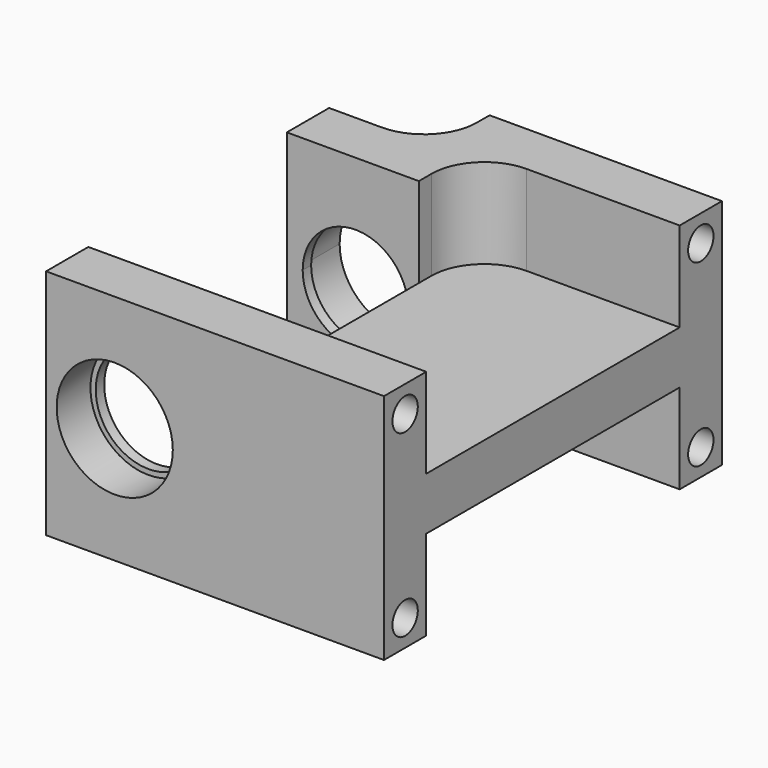
from build123d import *

# Parameters (mm, degrees)
F0_W      = 5
F0_H      = 5
F0_H_2    = 8.5
F0_W_2    = 30
F1_DEPTH  = 30
F2_DEPTH  = 2
F4_W      = 10.5
F4_H      = 30
F5_DEPTH  = 13.501
F3_R      = 5.5
F3_R_2    = 5
F3_R_3    = 2.5
F6_DEPTH  = 4
F7_DEPTH  = 5
F9_DEPTH  = 22
F10_DEPTH = 8
F11_DEPTH = 1.5
F12_R     = 5
F13_R     = 5
F15_DEPTH = 10.5
F14_R     = 2.5
F16_DEPTH = 11.5
F18_D     = 3
F20_D     = 2.5
F20_DEPTH = 15
F20_TIP   = 0.7510757738


# Not quite as in the source:
# - a feature names something its author has since deleted; it is built from what else it names


with BuildPart() as f1:
    # F0 (on Right) → F1 (new body)
    with BuildSketch(Plane.YZ):
        with Locations((17.5, 0)):
            Rectangle(F0_W, F0_H)
        with Locations((17.5, 6.75)):
            Rectangle(F0_W, F0_H_2)
        Rectangle(F0_W_2, F0_H)
        with Locations((17.5, -6.75)):
            Rectangle(F0_W, F0_H_2)
        with Locations((-17.5, 0)):
            Rectangle(F0_W, F0_H)
        with Locations((-17.5, 6.75)):
            Rectangle(F0_W, F0_H_2)
        with Locations((-17.5, -6.75)):
            Rectangle(F0_W, F0_H_2)
    extrude(amount=F1_DEPTH)

    # F0 (on Right) → F2 (join)
    with BuildSketch(Plane.YZ):
        with Locations((-17.5, 6.75)):
            Rectangle(F0_W, F0_H_2)
        with Locations((-17.5, 0)):
            Rectangle(F0_W, F0_H)
        with Locations((-17.5, -6.75)):
            Rectangle(F0_W, F0_H_2)
    extrude(amount=-F2_DEPTH)

    # F4 (on face) → F5 (cut, through all)
    with BuildSketch(Plane.XY.offset(2.5)):
        with Locations((5.25, 0)):
            Rectangle(F4_W, F4_H)
    extrude(amount=-F5_DEPTH, mode=Mode.SUBTRACT)

    # F3 (on face) → F6 (cut)
    with BuildSketch(Plane.XZ.offset(20)):
        with Locations((4.5, 0)):
            Circle(F3_R)
        with Locations((4.5, 0)):
            Circle(F3_R_2, mode=Mode.SUBTRACT)
        with Locations((4.5, 0)):
            Circle(F3_R_2)
        with Locations((4.5, 0)):
            Circle(F3_R_3, mode=Mode.SUBTRACT)
        with Locations((4.5, 0)):
            Circle(F3_R_3)
    extrude(amount=-F6_DEPTH, mode=Mode.SUBTRACT)

    # F3 (on face) → F7 (cut, through all)
    with BuildSketch(Plane.XZ.offset(20)):
        with Locations((4.5, 0)):
            Circle(F3_R_2)
        with Locations((4.5, 0)):
            Circle(F3_R_3, mode=Mode.SUBTRACT)
        with Locations((4.5, 0)):
            Circle(F3_R_3)
    extrude(amount=-F7_DEPTH, mode=Mode.SUBTRACT)

    # F8 (on face) → F9 (join, through all)
    with BuildSketch(Plane.XY.offset(11)):
        Polygon((10.5, 8.5), (10.5, 15), (0, 15), (-2, 15), (-2, 8.5), align=None)
    extrude(amount=-F9_DEPTH)

    # F10 (cut): a face of the model
    f10_faces = [f1.faces().sort_by_distance(p)[0] for p in [
        (0, 17.5, 0),
    ]]
    extrude(f10_faces, amount=-F10_DEPTH, mode=Mode.SUBTRACT)

    # F11 (cut): a face of the model
    f11_faces = [f1.faces().sort_by_distance(p)[0] for p in [
        (3, 15, 0),
    ]]
    extrude(f11_faces, amount=-F11_DEPTH, mode=Mode.SUBTRACT)

    # F12
    f12_edges = [f1.edges().sort_by_distance(p)[0] for p in [
        (8, 13.5, 0),
    ]]
    fillet(f12_edges, radius=F12_R)

    # F13
    f13_edges = [f1.edges().sort_by_distance(p)[0] for p in [
        (10.5, 15, 6.75),
        (10.5, 15, -6.75),
    ]]
    fillet(f13_edges, radius=F13_R)

    # F14 (on face) → F15 (cut)
    with BuildSketch(Plane(origin=(0, 20, 0), x_dir=(-1, 0, 0), z_dir=(0, 1, 0))):
        with BuildLine():
            Line((-8, 3.5707142143), (-8, 4.2426406871))
            ThreePointArc((-8, 4.2426406871), (-10, 0), (-8, -4.2426406871))
            Line((-8, -4.2426406871), (-8, -3.5707142143))
            ThreePointArc((-8, -3.5707142143), (-9.5, 0), (-8, 3.5707142143))
        make_face()
        with BuildLine():
            ThreePointArc((-8, -4.2426406871), (-2.1547921201, -4.9749371855), (1, 0))
            ThreePointArc((1, 0), (-2.1547921201, 4.9749371855), (-8, 4.2426406871))
            Line((-8, 4.2426406871), (-8, 3.5707142143))
            ThreePointArc((-8, 3.5707142143), (-2.5635083269, 4.6097722286), (0.5, 0))
            ThreePointArc((0.5, 0), (-2.5635083269, -4.6097722286), (-8, -3.5707142143))
            Line((-8, -3.5707142143), (-8, -4.2426406871))
        make_face()
    extrude(amount=-F15_DEPTH, mode=Mode.SUBTRACT)

    # F14 (on face) → F16 (cut, through all)
    with BuildSketch(Plane(origin=(0, 20, 0), x_dir=(-1, 0, 0), z_dir=(0, 1, 0))):
        with BuildLine():
            ThreePointArc((0.5, 0), (-2.5635083269, 4.6097722286), (-8, 3.5707142143))
            Line((-8, 3.5707142143), (-8, -3.5707142143))
            ThreePointArc((-8, -3.5707142143), (-2.5635083269, -4.6097722286), (0.5, 0))
        make_face()
        with Locations((-4.5, 0)):
            Circle(F14_R, mode=Mode.SUBTRACT)
        with Locations((-4.5, 0)):
            Circle(F14_R)
        with BuildLine():
            Line((-8, -3.5707142143), (-8, 3.5707142143))
            ThreePointArc((-8, 3.5707142143), (-9.5, 0), (-8, -3.5707142143))
        make_face()
    extrude(amount=-F16_DEPTH, mode=Mode.SUBTRACT)

    # F18 (through all)
    with Locations(Plane.YZ.offset(30)):
        with Locations((-17.5, 8.5), (-17.5, -8.5), (17.5, 8.5), (17.5, -8.5)):
            Hole(F18_D / 2)

    # F20
    with Locations(Plane(origin=(0, 20, 0), x_dir=(-1, 0, 0), z_dir=(0, 1, 0))):
        with Locations((-25, 0)):
            Hole(F20_D / 2, depth=F20_DEPTH)
            with Locations((0, 0, -(F20_DEPTH + F20_TIP / 2))):  # 118° drill point
                Cone(0, F20_D / 2, F20_TIP, mode=Mode.SUBTRACT)


solid = f1.part
